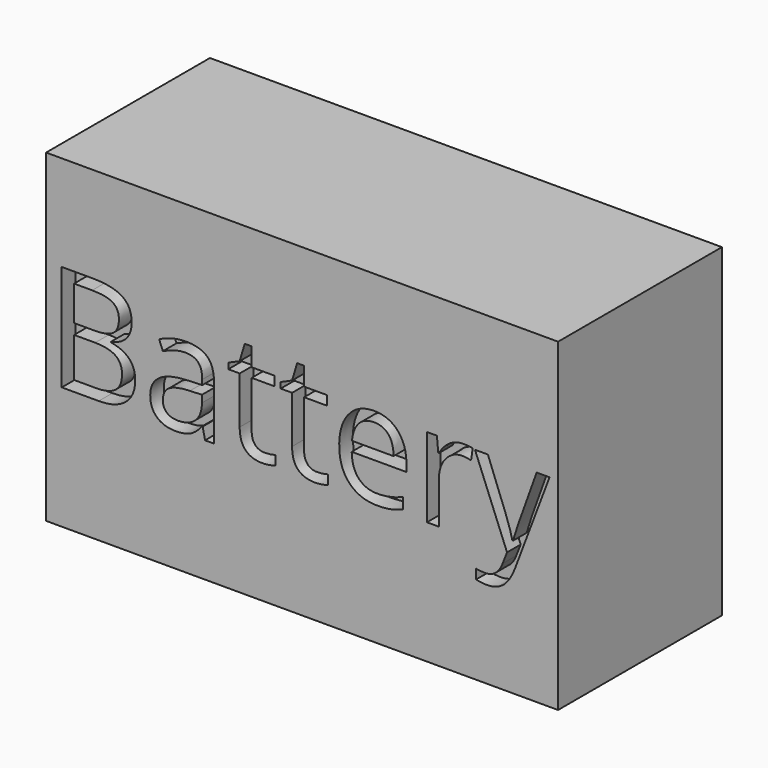
from build123d import *

# Parameters (mm, degrees)
F0_W         = 150
F0_H         = 95
F1_DEPTH     = 60
F2_TEXT_SIZE = 43.5137340223
F3_DEPTH     = 5


# Not quite as in the source:
# - Text() gives the source's letters only with a copy of the font that has no kerning and outlines rounded to 1/6400 em; it was checked with that copy


with BuildPart() as f1:
    # F0 (on Front) → F1 (new body)
    with BuildSketch(Plane.XZ):
        Rectangle(F0_W, F0_H)
    extrude(amount=F1_DEPTH)

    # F2 (on face) → F3 (cut)
    with BuildSketch(Plane.XZ.offset(60)):
        with Locations((-74.6795935142, -11.5719165582)):
            Text('Battery', F2_TEXT_SIZE, font='Open Sans', text_align=(TextAlign.LEFT, TextAlign.BOTTOM))
    extrude(amount=-F3_DEPTH, mode=Mode.SUBTRACT)


solid = f1.part
